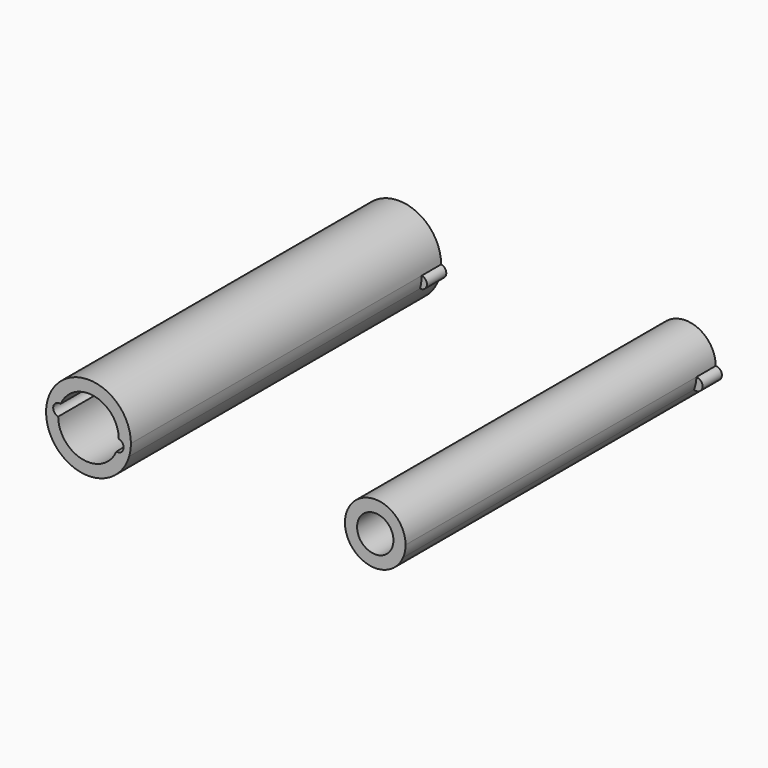
from build123d import *

# Parameters (mm, degrees)
F0_R     = 2.38125
F1_DEPTH = 50.8
F2_DEPTH = 3.175
F3_DEPTH = 3.175


# Not quite as in the source:
# - a feature names something its author has since deleted; it is built from what else it names


with BuildPart() as f1:
    # F0 (on Front) → F1 (new body)
    with BuildSketch(Plane.XZ):
        with BuildLine():
            ThreePointArc((49.9514526081, -1.5554259867), (50.1887675748, -0.79375), (50.2689526081, 0))
            ThreePointArc((50.2689526081, 0), (47.0939526081, 3.8885649667), (42.6489526081, 1.5554259867))
            ThreePointArc((42.6489526081, 1.5554259867), (42.4116376414, 0.79375), (42.3314526081, 0))
            ThreePointArc((42.3314526081, 0), (45.5064526081, -3.8885649667), (49.9514526081, -1.5554259867))
        make_face()
        with Locations((46.3002026081, 0)):
            Circle(F0_R, mode=Mode.SUBTRACT)
    extrude(amount=F1_DEPTH)

    # F0 (on Front) → F3 (join)
    with BuildSketch(Plane.XZ):
        with BuildLine():
            ThreePointArc((49.9514526081, -1.5554259867), (51.0627026081, -0.9721412417), (50.2689526081, 0))
            ThreePointArc((50.2689526081, 0), (50.1887675748, -0.79375), (49.9514526081, -1.5554259867))
        make_face()
        with BuildLine():
            ThreePointArc((42.3314526081, 0), (42.4116376414, 0.79375), (42.6489526081, 1.5554259867))
            ThreePointArc((42.6489526081, 1.5554259867), (41.654489723, 0.9483021717), (42.3314526081, 0))
        make_face()
    extrude(amount=F3_DEPTH)


with BuildPart() as f1b:
    # F0 (on Front) → F1, piece 2 (new body)
    with BuildSketch(Plane.XZ):
        with BuildLine():
            ThreePointArc((14.0615205309, -1.5712175183), (14.2313175592, -0.79375), (14.2883062452, 0))
            ThreePointArc((14.2883062452, 0), (9.534209736, 5.4980418187), (3.4074193738, 1.5875))
            ThreePointArc((3.4074193738, 1.5875), (3.2340144266, 0.8021534908), (3.1758062452, 0))
            ThreePointArc((3.1758062452, 0), (7.9383062452, -5.499261314), (14.0615205309, -1.5712175183))
        make_face()
        with BuildLine():
            ThreePointArc((5.0946367873, 1.5875), (9.5429101436, 3.8850344294), (12.7008062452, 0))
            ThreePointArc((12.7008062452, 0), (13.3197692385, -0.9364629933), (12.3833062452, -1.5554259867))
            ThreePointArc((12.3833062452, -1.5554259867), (7.9383062452, -3.8885649667), (4.7633062452, 0))
            ThreePointArc((4.7633062452, 0), (4.1277289023, 0.9609790707), (5.0946367873, 1.5875))
        make_face(mode=Mode.SUBTRACT)
    extrude(amount=F1_DEPTH)


with BuildPart() as f2:
    # F0 (on Front) → F2 (new body)
    with BuildSketch(Plane.XZ):
        with BuildLine():
            ThreePointArc((4.7633062452, 0), (4.8470218158, 0.8108538984), (5.0946367873, 1.5875))
            ThreePointArc((5.0946367873, 1.5875), (4.1277289023, 0.9609790707), (4.7633062452, 0))
        make_face()
    extrude(amount=F2_DEPTH)


with BuildPart() as f2b:
    # F0 (on Front) → F2, piece 2 (new body)
    with BuildSketch(Plane.XZ):
        with BuildLine():
            ThreePointArc((12.3833062452, -1.5554259867), (13.3197692385, -0.9364629933), (12.7008062452, 0))
            ThreePointArc((12.7008062452, 0), (12.6206212119, -0.79375), (12.3833062452, -1.5554259867))
        make_face()
    extrude(amount=F2_DEPTH)


with BuildPart() as f2c:
    # F0 (on Front) → F2, piece 3 (new body)
    with BuildSketch(Plane.XZ):
        with BuildLine():
            ThreePointArc((14.0615205309, -1.5712175183), (14.9605221472, -0.8990016163), (14.2883062452, 0))
            ThreePointArc((14.2883062452, 0), (14.2313175592, -0.79375), (14.0615205309, -1.5712175183))
        make_face()
    extrude(amount=F2_DEPTH)


with BuildPart() as f2d:
    # F0 (on Front) → F2, piece 4 (new body)
    with BuildSketch(Plane.XZ):
        with BuildLine():
            ThreePointArc((3.1758062452, 0), (3.2340144266, 0.8021534908), (3.4074193738, 1.5875))
            ThreePointArc((3.4074193738, 1.5875), (2.6170785878, 0.8921632166), (3.1758062452, 0))
        make_face()
    extrude(amount=F2_DEPTH)


solid = Compound([f1.part, f1b.part, f2.part, f2b.part, f2c.part, f2d.part])
